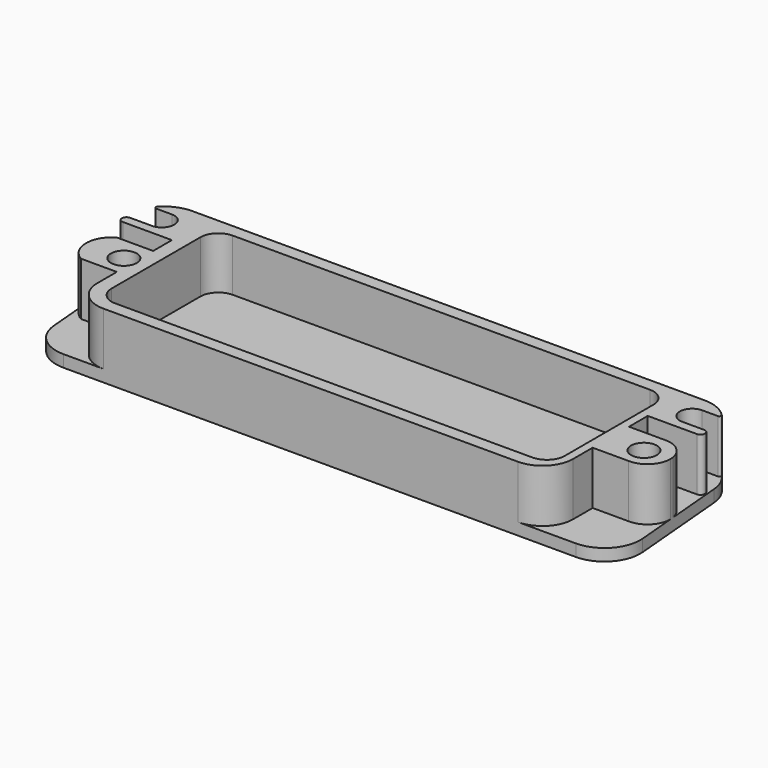
from build123d import *

# Parameters (mm, degrees)
F1_DEPTH       = 17.272
F3_DEPTH       = 13.843
F5_DEPTH       = 14.097
F7_D           = 6.858
F7_CBORE_D     = 10.033
F7_CBORE_DEPTH = 3.048


# Not quite as in the source:
# - a feature names something its author has since deleted; it is built from what else it names


with BuildPart() as f1:
    # F0 (on Top) → F1 (new body)
    with BuildSketch(Plane.XY):
        with BuildLine():
            Line((68.0447455007, 22.86), (-68.0447455007, 22.86))
            ThreePointArc((-68.0447455007, 22.86), (-75.0673121338, 19.7699967275), (-77.5335, 12.5048415503))
            Line((-77.5335, 12.5048415503), (-75.2001773438, -14.1651584497))
            ThreePointArc((-75.2001773438, -14.1651584497), (-72.146419572, -20.3575666331), (-65.7114228444, -22.86))
            Line((-65.7114228444, -22.86), (70.3780681569, -22.86))
            ThreePointArc((70.3780681569, -22.86), (77.40063479, -19.7699967275), (79.8668226562, -12.5048415503))
            Line((79.8668226562, -12.5048415503), (77.5335, 14.1651584497))
            ThreePointArc((77.5335, 14.1651584497), (74.4797422282, 20.3575666331), (68.0447455007, 22.86))
        make_face()
    extrude(amount=F1_DEPTH)

    # F2 (on face) → F3 (cut)
    with BuildSketch(Plane.XY.offset(17.272)):
        with BuildLine():
            Line((56.1975, 19.4945), (-54.61, 19.4945))
            ThreePointArc((-54.61, 19.4945), (-57.9775960454, 18.0995960454), (-59.3725, 14.732))
            Line((-59.3725, 14.732), (-59.3725, -14.732))
            ThreePointArc((-59.3725, -14.732), (-57.9775960454, -18.0995960454), (-54.61, -19.4945))
            Line((-54.61, -19.4945), (56.1975, -19.4945))
            ThreePointArc((56.1975, -19.4945), (59.5650960454, -18.0995960454), (60.96, -14.732))
            Line((60.96, -14.732), (60.96, 14.732))
            ThreePointArc((60.96, 14.732), (59.5650960454, 18.0995960454), (56.1975, 19.4945))
        make_face()
    extrude(amount=-F3_DEPTH, mode=Mode.SUBTRACT)

    # F4 (on face) → F5 (cut)
    with BuildSketch(Plane.XY.offset(17.272)):
        with BuildLine():
            Line((-76.239581844, -2.2847106486), (-77.4044675129, 11.0299934736))
            ThreePointArc((-77.4044675129, 11.0299934736), (-77.4182058621, 11.1343465964), (-77.4227969589, 11.2395))
            Line((-77.4227969589, 11.2395), (-77.5335, 12.5048415503))
            ThreePointArc((-77.5335, 12.5048415503), (-77.0333154818, 16.4863861544), (-74.9377505887, 19.9085915493))
            ThreePointArc((-74.9377505887, 19.9085915493), (-71.7938897692, 22.0911145638), (-68.0447455007, 22.86))
            Line((-68.0447455007, 22.86), (-80.5285722017, 22.86))
            Line((-80.5285722017, 22.86), (-80.5285722017, -22.86))
            Line((-80.5285722017, -22.86), (-65.7114228444, -22.86))
            ThreePointArc((-65.7114228444, -22.86), (-72.146419572, -20.3575666331), (-75.2001773438, -14.1651584497))
            Line((-75.2001773438, -14.1651584497), (-76.1550120261, -3.2513480896))
            ThreePointArc((-76.1550120261, -3.2513480896), (-76.2140031856, -2.7694909766), (-76.239581844, -2.2847106486))
        make_face()
        with BuildLine():
            Line((-77.5335, 12.5048415503), (-77.4227969589, 11.2395))
            ThreePointArc((-77.4227969589, 11.2395), (-77.0694212904, 12.0926243315), (-76.2162969589, 12.446))
            Line((-76.2162969589, 12.446), (-70.4215, 12.446))
            ThreePointArc((-70.4215, 12.446), (-67.1195, 15.748), (-70.4215, 19.05))
            Line((-70.4215, 19.05), (-74.5701236506, 19.05))
            ThreePointArc((-74.5701236506, 19.05), (-75.0371164274, 19.358045639), (-74.9377505887, 19.9085915493))
            ThreePointArc((-74.9377505887, 19.9085915493), (-77.0333154818, 16.4863861544), (-77.5335, 12.5048415503))
        make_face()
        with BuildLine():
            Line((-63.1825, 3.81), (-63.1825, 10.033))
            Line((-63.1825, 10.033), (-76.2162969589, 10.033))
            ThreePointArc((-76.2162969589, 10.033), (-76.9918202099, 10.3152673794), (-77.4044675129, 11.0299934736))
            Line((-77.4044675129, 11.0299934736), (-76.239581844, -2.2847106486))
            ThreePointArc((-76.239581844, -2.2847106486), (-75.3866698867, 1.2003753653), (-72.9243249481, 3.81))
            Line((-72.9243249481, 3.81), (-63.1825, 3.81))
        make_face()
        with BuildLine():
            ThreePointArc((-72.7051694123, -8.255), (-74.9990780637, -6.1454708758), (-76.1550120261, -3.2513480896))
            Line((-76.1550120261, -3.2513480896), (-75.2001773438, -14.1651584497))
            ThreePointArc((-75.2001773438, -14.1651584497), (-72.146419572, -20.3575666331), (-65.7114228444, -22.86))
            Line((-65.7114228444, -22.86), (-55.0545, -22.86))
            ThreePointArc((-55.0545, -22.86), (-60.8018639175, -20.4793639175), (-63.1825, -14.732))
            Line((-63.1825, -14.732), (-63.1825, -8.255))
            Line((-63.1825, -8.255), (-72.7051694123, -8.255))
        make_face()
        with BuildLine():
            ThreePointArc((63.1825, -14.732), (60.8018639175, -20.4793639175), (55.0545, -22.86))
            Line((55.0545, -22.86), (70.3780681569, -22.86))
            ThreePointArc((70.3780681569, -22.86), (77.40063479, -19.7699967275), (79.8668226562, -12.5048415503))
            Line((79.8668226562, -12.5048415503), (78.9578200825, -2.114894589))
            ThreePointArc((78.9578200825, -2.114894589), (77.1524285249, -6.5300931701), (72.7051694123, -8.255))
            Line((72.7051694123, -8.255), (63.1825, -8.255))
            Line((63.1825, -8.255), (63.1825, -14.732))
        make_face()
        with BuildLine():
            ThreePointArc((77.5335, 14.1651584497), (76.7244498583, 17.2577996716), (74.9377505887, 19.9085915493))
            ThreePointArc((74.9377505887, 19.9085915493), (75.0371164274, 19.358045639), (74.5701236506, 19.05))
            Line((74.5701236506, 19.05), (70.4215, 19.05))
            ThreePointArc((70.4215, 19.05), (67.1195, 15.748), (70.4215, 12.446))
            Line((70.4215, 12.446), (76.2162969589, 12.446))
            ThreePointArc((76.2162969589, 12.446), (77.4227969589, 11.2395), (76.2162969589, 10.033))
            Line((76.2162969589, 10.033), (63.1825, 10.033))
            Line((63.1825, 10.033), (63.1825, 3.81))
            Line((63.1825, 3.81), (72.9243249481, 3.81))
            ThreePointArc((72.9243249481, 3.81), (76.8450400591, 2.3627819378), (78.8851888528, -1.2847158349))
            Line((78.8851888528, -1.2847158349), (77.5335, 14.1651584497))
        make_face()
    extrude(amount=-F5_DEPTH, mode=Mode.SUBTRACT)

    # F7 (through all)
    with Locations(Plane(origin=(0, 0, 0), x_dir=(1, 0, 0), z_dir=(0, 0, -1))):
        with Locations((72.23125, 2.54), (-65.88125, 2.54)):
            CounterBoreHole(F7_D / 2, F7_CBORE_D / 2, F7_CBORE_DEPTH)


solid = f1.part
